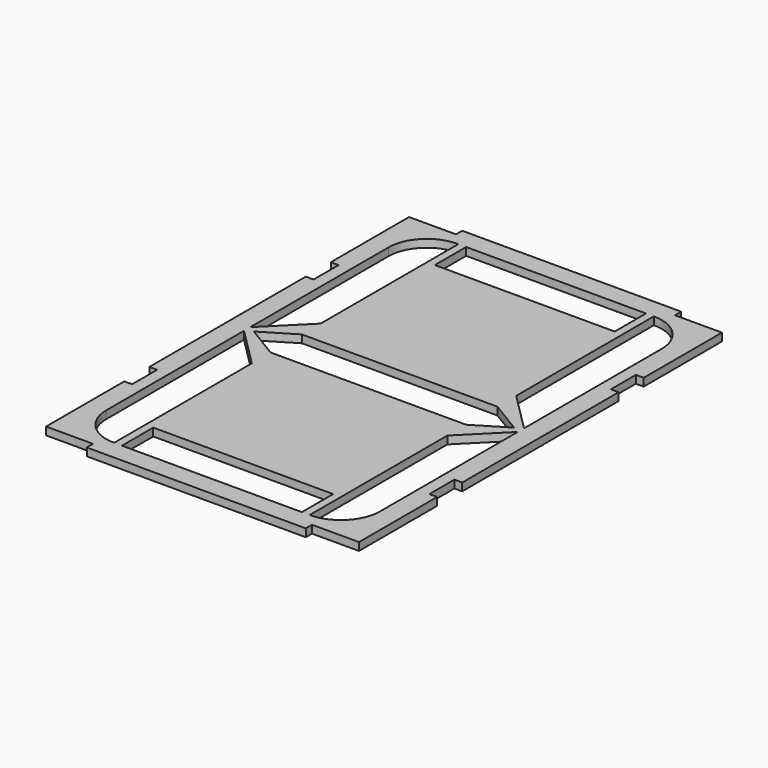
from build123d import *

# Parameters (mm, degrees)
F0_W      = 101.6
F0_H      = 152.4
F1_DEPTH  = 2.54
F2_W      = 12.7
F2_H      = 68.58
F3_DEPTH  = 2.541
F4_SIZE2  = 12.69999
F4_SIZE   = 12.69999
F5_R      = 12.446
F6_W      = 58.42
F6_H      = 12.7
F7_DEPTH  = 2.541
F8_W      = 12.7
F8_H      = 68.58
F9_DEPTH  = 2.541
F10_R     = 12.69999
F11_SIZE2 = 12.69999
F11_SIZE  = 12.69999
F12_W     = 12.7
F12_H     = 68.58
F13_DEPTH = 2.541
F14_SIZE2 = 12.69999
F14_SIZE  = 12.69999
F15_R     = 12.69999
F16_W     = 12.7
F16_H     = 68.58
F17_DEPTH = 2.541
F18_SIZE2 = 12.69999
F18_SIZE  = 12.69999
F19_R     = 12.69999
F20_W     = 58.42
F20_H     = 12.7
F21_DEPTH = 2.541
F23_DEPTH = 25.4
F25_DEPTH = 25.4
F27_DEPTH = 25.4
F28_W     = 2.54
F28_H     = 10.16
F29_DEPTH = 25.4
F30_W     = 2.54
F30_H     = 10.16
F31_DEPTH = 25.4
F32_W     = 15.24
F32_H     = 2.54
F33_DEPTH = 25.4


# Not quite as in the source:
# - a fillet or chamfer is up to 0.001 mm smaller than in the source, because OpenCascade refuses the exact size


with BuildPart() as f1:
    # F0 (on Top) → F1 (new body)
    with BuildSketch(Plane.XY):
        Rectangle(F0_W, F0_H)
    extrude(amount=F1_DEPTH)

    # F2 (on face) → F3 (cut, through all)
    with BuildSketch(Plane.XY.offset(2.54)):
        with Locations((-38.1, 35.56)):
            Rectangle(F2_W, F2_H)
    extrude(amount=-F3_DEPTH, mode=Mode.SUBTRACT)

    # F4 (size 12.7 and 12.7 in the source; OpenCascade refuses exactly that, so slightly less here)
    f4_edges = [f1.edges().sort_by_distance(p)[0] for p in [
        (-31.75, 1.27, 1.27),
    ]]
    chamfer(f4_edges, length=F4_SIZE, length2=F4_SIZE2)

    # F5
    f5_edges = [f1.edges().sort_by_distance(p)[0] for p in [
        (-44.45, 69.85, 1.27),
    ]]
    fillet(f5_edges, radius=F5_R)

    # F6 (on face) → F7 (cut, through all)
    with BuildSketch(Plane.XY.offset(2.54)):
        with Locations((0, 63.5)):
            Rectangle(F6_W, F6_H)
    extrude(amount=-F7_DEPTH, mode=Mode.SUBTRACT)

    # F8 (on face) → F9 (cut, through all)
    with BuildSketch(Plane.XY.offset(2.54)):
        with Locations((38.1, 35.56)):
            Rectangle(F8_W, F8_H)
    extrude(amount=-F9_DEPTH, mode=Mode.SUBTRACT)

    # F10 (radius 12.7 in the source; OpenCascade refuses exactly that, so slightly less here)
    f10_edges = [f1.edges().sort_by_distance(p)[0] for p in [
        (44.45, 69.85, 1.27),
    ]]
    fillet(f10_edges, radius=F10_R)

    # F11 (size 12.7 and 12.7 in the source; OpenCascade refuses exactly that, so slightly less here)
    f11_edges = [f1.edges().sort_by_distance(p)[0] for p in [
        (31.75, 1.27, 1.27),
    ]]
    chamfer(f11_edges, length=F11_SIZE, length2=F11_SIZE2)

    # F12 (on face) → F13 (cut, through all)
    with BuildSketch(Plane.XY.offset(2.54)):
        with Locations((-38.1, -35.56)):
            Rectangle(F12_W, F12_H)
    extrude(amount=-F13_DEPTH, mode=Mode.SUBTRACT)

    # F14 (size 12.7 and 12.7 in the source; OpenCascade refuses exactly that, so slightly less here)
    f14_edges = [f1.edges().sort_by_distance(p)[0] for p in [
        (-31.75, -1.27, 1.27),
    ]]
    chamfer(f14_edges, length=F14_SIZE, length2=F14_SIZE2)

    # F15 (radius 12.7 in the source; OpenCascade refuses exactly that, so slightly less here)
    f15_edges = [f1.edges().sort_by_distance(p)[0] for p in [
        (-44.45, -69.85, 1.27),
    ]]
    fillet(f15_edges, radius=F15_R)

    # F16 (on face) → F17 (cut, through all)
    with BuildSketch(Plane.XY.offset(2.54)):
        with Locations((38.1, -35.56)):
            Rectangle(F16_W, F16_H)
    extrude(amount=-F17_DEPTH, mode=Mode.SUBTRACT)

    # F18 (size 12.7 and 12.7 in the source; OpenCascade refuses exactly that, so slightly less here)
    f18_edges = [f1.edges().sort_by_distance(p)[0] for p in [
        (31.75, -1.27, 1.27),
    ]]
    chamfer(f18_edges, length=F18_SIZE, length2=F18_SIZE2)

    # F19 (radius 12.7 in the source; OpenCascade refuses exactly that, so slightly less here)
    f19_edges = [f1.edges().sort_by_distance(p)[0] for p in [
        (44.45, -69.85, 1.27),
    ]]
    fillet(f19_edges, radius=F19_R)

    # F20 (on face) → F21 (cut, through all)
    with BuildSketch(Plane.XY.offset(2.54)):
        with Locations((0, -63.5)):
            Rectangle(F20_W, F20_H)
    extrude(amount=-F21_DEPTH, mode=Mode.SUBTRACT)

    # F22 (on face) → F23 (cut)
    with BuildSketch(Plane.XY.offset(2.54)):
        Polygon((-31.75, 6.35), (-42.2502954744, 0), (-31.75, -6.35), (31.75, -6.35), (42.2502954744, 0), (31.75, 6.35), align=None)
    extrude(amount=-F23_DEPTH, mode=Mode.SUBTRACT)

    # F24 (on face) → F25 (cut)
    with BuildSketch(Plane.XY.offset(2.54)):
        Polygon((-50.8, -76.2), (-39.37, -76.2), (-41.91, -73.66), (-50.8, -73.66), align=None)
        Polygon((41.91, -73.66), (39.37, -76.2), (50.8, -76.2), (50.8, -73.66), align=None)
    extrude(amount=-F25_DEPTH, mode=Mode.SUBTRACT)

    # F26 (on face) → F27 (cut)
    with BuildSketch(Plane.XY.offset(2.54)):
        Polygon((-39.37, 76.2), (-50.8, 76.2), (-50.8, 73.66), (-41.91, 73.66), align=None)
        Polygon((50.8, 76.2), (39.37, 76.2), (41.91, 73.66), (50.8, 73.66), align=None)
    extrude(amount=-F27_DEPTH, mode=Mode.SUBTRACT)

    # F28 (on face) → F29 (cut)
    with BuildSketch(Plane.XY.offset(2.54)):
        with Locations((49.53, 36.83)):
            Rectangle(F28_W, F28_H)
        with Locations((49.53, -36.83)):
            Rectangle(F28_W, F28_H)
    extrude(amount=-F29_DEPTH, mode=Mode.SUBTRACT)

    # F30 (on face) → F31 (cut)
    with BuildSketch(Plane.XY.offset(2.54)):
        with Locations((-49.53, 36.83)):
            Rectangle(F30_W, F30_H)
        with Locations((-49.53, -36.83)):
            Rectangle(F30_W, F30_H)
    extrude(amount=-F31_DEPTH, mode=Mode.SUBTRACT)

    # F32 (on face) → F33 (cut)
    with BuildSketch(Plane.XY.offset(2.54)):
        with Locations((-43.18, -74.93)):
            Rectangle(F32_W, F32_H)
        with Locations((43.18, -74.93)):
            Rectangle(F32_W, F32_H)
        with Locations((-43.18, 74.93)):
            Rectangle(F32_W, F32_H)
        with Locations((43.18, 74.93)):
            Rectangle(F32_W, F32_H)
    extrude(amount=-F33_DEPTH, mode=Mode.SUBTRACT)


solid = f1.part
